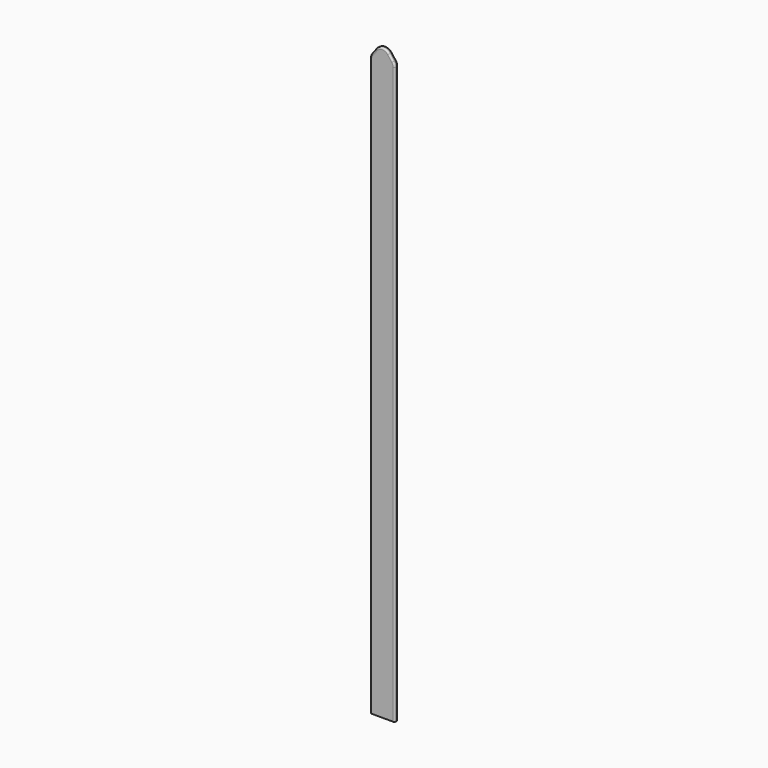
from build123d import *

# Parameters (mm, degrees)
F1_DEPTH     = 3.175
F2_R         = 2.54
F3_T1_DEPTH  = 6.35
F3_T4_ANGLE  = 36.869898
F3_T6_ANGLE  = 106.260205
F3_T8_ANGLE  = 36.869898
F3_T10_ANGLE = 36.869898
F3_T12_ANGLE = 106.260205
F3_T14_ANGLE = 36.869898


# Not quite as in the source:
# - a fillet or chamfer that OpenCascade refuses, or shapes differently, is made with other operations: its cross-section is extruded or revolved along the edge and cut away or added


with BuildPart() as f1:
    # F0 (on Front) → F1 (new body, symmetric)
    with BuildSketch(Plane.XZ):
        Polygon((-19.05, 889), (-19.05, 0), (19.05, 0), (19.05, 889), (0, 914.4), align=None)
    extrude(amount=F1_DEPTH, both=True)

    # F2
    f2_edges = [f1.edges().sort_by_distance(p)[0] for p in [
        (-19.05, -3.175, 444.5),
        (-19.05, 3.175, 444.5),
        (-9.525, -3.175, 901.7),
        (9.525, -3.175, 901.7),
        (19.05, -3.175, 444.5),
        (19.05, 3.175, 444.5),
        (9.525, 3.175, 901.7),
        (-9.525, 3.175, 901.7),
    ]]
    fillet(f2_edges, radius=F2_R)

    # F3: fillet of radius 12.7 on 3 edges, made by hand

    # F3_s2 → F3_t1 (cut)
    with BuildSketch(Plane.XZ.offset(-3.175)):
        with BuildLine():
            ThreePointArc((19.05, 884.766667), (18.398278, 888.782759), (16.51, 892.386667))
            Line((16.51, 892.386667), (19.05, 889))
            Line((19.05, 889), (19.05, 884.766667))
        make_face()
        with BuildLine():
            ThreePointArc((-10.16, 900.853333), (0, 905.933333), (10.16, 900.853333))
            Line((10.16, 900.853333), (0, 914.4))
            Line((0, 914.4), (-10.16, 900.853333))
        make_face()
        with BuildLine():
            ThreePointArc((-19.05, 884.766667), (-18.398278, 888.782759), (-16.51, 892.386667))
            Line((-16.51, 892.386667), (-19.05, 889))
            Line((-19.05, 889), (-19.05, 884.766667))
        make_face()
    extrude(amount=F3_T1_DEPTH, mode=Mode.SUBTRACT)

    # F3_s3 → F3_t4 (revolve, cut)
    with BuildSketch(Plane(origin=(422.402, 0, 563.202667), x_dir=(0, 1, 0), z_dir=(0.6, 0, 0.8))):
        with BuildLine():
            ThreePointArc((-3.175, 546.1), (-2.431051, 547.896051), (-0.635, 548.64))
            Line((-0.635, 548.64), (-3.175, 548.64))
            Line((-3.175, 548.64), (-3.175, 546.1))
        make_face()
    revolve(axis=Axis((-6.35, -3.175, 884.766667), (0, -1, 0)), revolution_arc=F3_T4_ANGLE, mode=Mode.SUBTRACT)

    # F3_s5 → F3_t6 (revolve, cut)
    with BuildSketch(Plane(origin=(-428.752, 0, 571.669333), x_dir=(0, 1, 0), z_dir=(0.6, 0, -0.8))):
        with BuildLine():
            ThreePointArc((-3.175, 546.1), (-2.431051, 547.896051), (-0.635, 548.64))
            Line((-0.635, 548.64), (-3.175, 548.64))
            Line((-3.175, 548.64), (-3.175, 546.1))
        make_face()
    revolve(axis=Axis((0, -3.175, 893.233333), (0, -1, 0)), revolution_arc=F3_T6_ANGLE, mode=Mode.SUBTRACT)

    # F3_s7 → F3_t8 (revolve, cut)
    with BuildSketch(Plane.XY.offset(884.766667)):
        with BuildLine():
            ThreePointArc((16.51, -3.175), (18.306051, -2.431051), (19.05, -0.635))
            Line((19.05, -0.635), (19.05, -3.175))
            Line((19.05, -3.175), (16.51, -3.175))
        make_face()
    revolve(axis=Axis((6.35, -3.175, 884.766667), (0, -1, 0)), revolution_arc=F3_T8_ANGLE, mode=Mode.SUBTRACT)

    # F3_s9 → F3_t10 (revolve, cut)
    with BuildSketch(Plane(origin=(-422.402, 0, 563.202667), x_dir=(0, 1, 0), z_dir=(-0.6, 0, 0.8))):
        with BuildLine():
            ThreePointArc((3.175, -546.1), (2.431051, -547.896051), (0.635, -548.64))
            Line((0.635, -548.64), (3.175, -548.64))
            Line((3.175, -548.64), (3.175, -546.1))
        make_face()
    revolve(axis=Axis((6.35, 3.175, 884.766667), (0, 1, 0)), revolution_arc=F3_T10_ANGLE, mode=Mode.SUBTRACT)

    # F3_s11 → F3_t12 (revolve, cut)
    with BuildSketch(Plane(origin=(428.752, 0, 571.669333), x_dir=(0, 1, 0), z_dir=(-0.6, 0, -0.8))):
        with BuildLine():
            ThreePointArc((3.175, -546.1), (2.431051, -547.896051), (0.635, -548.64))
            Line((0.635, -548.64), (3.175, -548.64))
            Line((3.175, -548.64), (3.175, -546.1))
        make_face()
    revolve(axis=Axis((0, 3.175, 893.233333), (0, 1, 0)), revolution_arc=F3_T12_ANGLE, mode=Mode.SUBTRACT)

    # F3_s13 → F3_t14 (revolve, cut)
    with BuildSketch(Plane.XY.offset(884.766667)):
        with BuildLine():
            ThreePointArc((-16.51, 3.175), (-18.306051, 2.431051), (-19.05, 0.635))
            Line((-19.05, 0.635), (-19.05, 3.175))
            Line((-19.05, 3.175), (-16.51, 3.175))
        make_face()
    revolve(axis=Axis((-6.35, 3.175, 884.766667), (0, 1, 0)), revolution_arc=F3_T14_ANGLE, mode=Mode.SUBTRACT)


solid = f1.part
